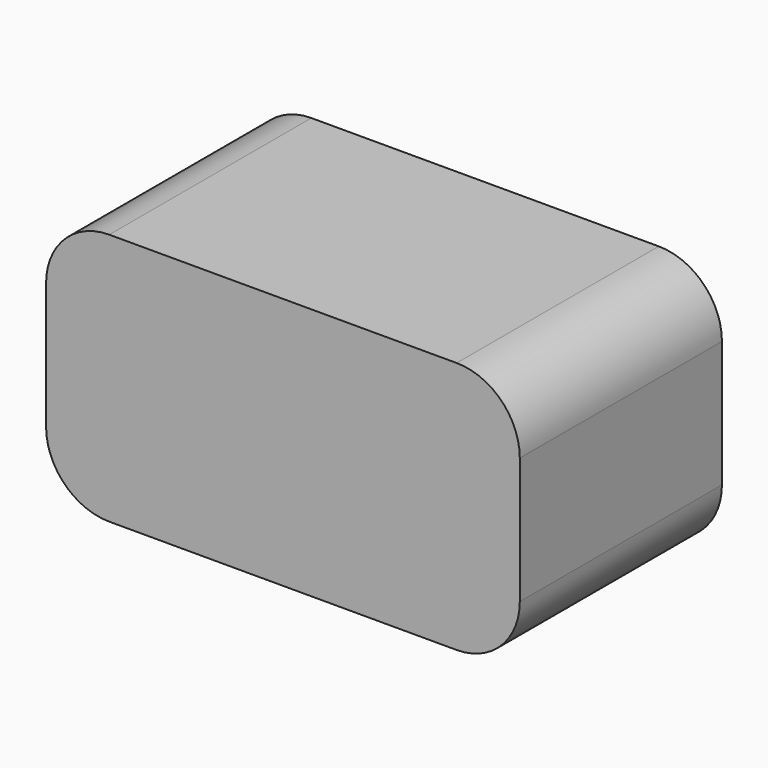
from build123d import *

# Parameters (mm, degrees)
F0_W     = 7.5
F0_H     = 4
F1_DEPTH = 2
F2_R     = 1


with BuildPart() as f1:
    # F0 (on Front) → F1 (new body, symmetric)
    with BuildSketch(Plane.XZ):
        Rectangle(F0_W, F0_H)
    extrude(amount=F1_DEPTH, both=True)

    # F2
    f2_edges = [f1.edges().sort_by_distance(p)[0] for p in [
        (-3.75, 0, 2),
        (-3.75, 0, -2),
        (3.75, 0, 2),
        (3.75, 0, -2),
    ]]
    fillet(f2_edges, radius=F2_R)


solid = f1.part
